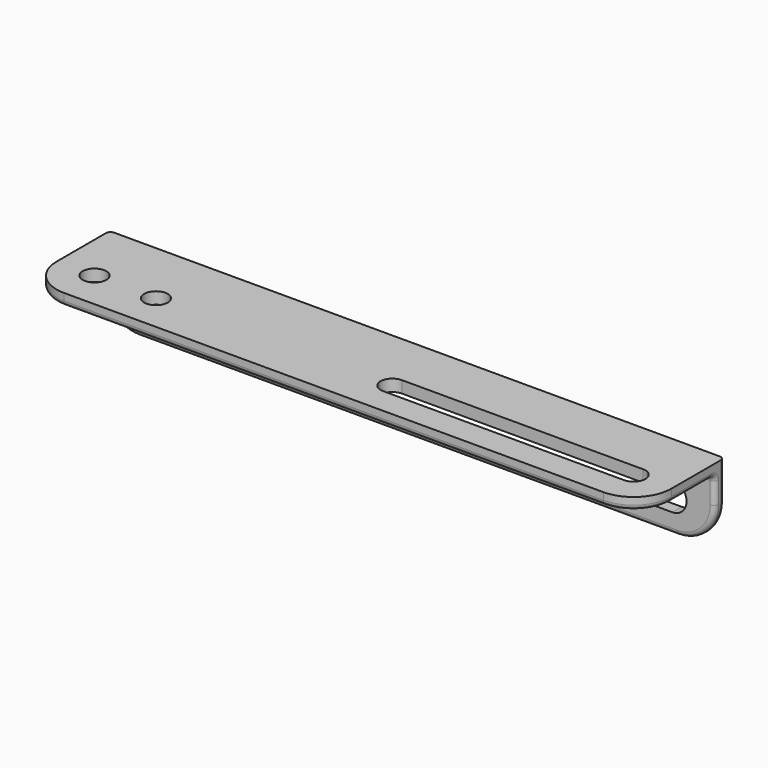
from build123d import *

# Parameters (mm, degrees)
F0_R     = 5
F1_DEPTH = 5
F2_W     = 260
F2_H     = 5
F3_DEPTH = 27
F4_R     = 16
F6_DEPTH = 5
F7_R     = 2


with BuildPart() as f1:
    # F0 (on Top) → F1 (new body)
    with BuildSketch(Plane.XY):
        with BuildLine():
            Line((130, -28), (130, 0))
            Line((130, 0), (-130, 0))
            Line((-130, 0), (-130, -28))
            ThreePointArc((-130, -28), (-125.313708499, -39.313708499), (-114, -44))
            Line((-114, -44), (114, -44))
            ThreePointArc((114, -44), (125.313708499, -39.313708499), (130, -28))
        make_face()
        with Locations((-114, -28)):
            Circle(F0_R, mode=Mode.SUBTRACT)
        with Locations((-88, -28)):
            Circle(F0_R, mode=Mode.SUBTRACT)
        with BuildLine():
            Line((12, -23), (114, -23))
            ThreePointArc((114, -23), (119, -28), (114, -33))
            Line((114, -33), (12, -33))
            ThreePointArc((12, -33), (7, -28), (12, -23))
        make_face(mode=Mode.SUBTRACT)
    extrude(amount=-F1_DEPTH)

    # F2 (on face) → F3 (join)
    with BuildSketch(Plane(origin=(0, 0, -5), x_dir=(1, 0, 0), z_dir=(0, 0, -1))):
        with Locations((0, 2.5)):
            Rectangle(F2_W, F2_H)
    extrude(amount=F3_DEPTH)

    # F4
    f4_edges = [f1.edges().sort_by_distance(p)[0] for p in [
        (130, -2.5, -32),
        (-130, -2.5, -32),
    ]]
    fillet(f4_edges, radius=F4_R)

    # F5 (on face) → F6 (cut)
    with BuildSketch(Plane(origin=(0, 0, 0), x_dir=(-1, 0, 0), z_dir=(0, 1, 0))):
        with BuildLine():
            ThreePointArc((48, -24), (54, -18), (48, -12))
            Line((48, -12), (-112, -12))
            ThreePointArc((-112, -12), (-118, -18), (-112, -24))
            Line((-112, -24), (48, -24))
        make_face()
    extrude(amount=-F6_DEPTH, mode=Mode.SUBTRACT)

    # F7
    f7_edges = [f1.edges().sort_by_distance(p)[0] for p in [
        (0, 0, -32),
        (-125.313708, -5, -27.313708),
        (0, -5, -5),
        (130, -5, -10.5),
        (130, -16.5, -5),
        (130, 0, -8),
        (125.313708, -5, -27.313708),
        (0, -5, -32),
        (-130, -5, -10.5),
        (125.313708, 0, -27.313708),
        (125.313708, -39.313708, -5),
        (0, -44, -5),
        (-125.313708, -39.313708, -5),
        (-130, -16.5, -5),
        (-130, 0, -8),
        (-125.313708, 0, -27.313708),
    ]]
    fillet(f7_edges, radius=F7_R)


solid = f1.part
